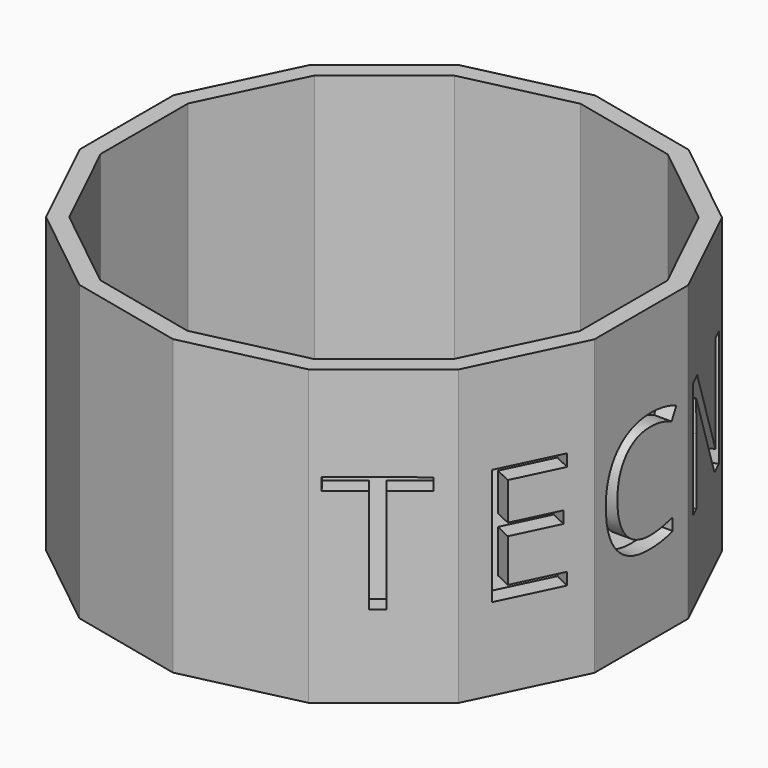
from build123d import *

# Parameters (mm, degrees)
F4_T          = -3
F5_TEXT_SIZE  = 27.7777777778
F6_DEPTH      = 25
F7_TEXT_SIZE  = 27.7777777778
F8_DEPTH      = 25
F9_TEXT_SIZE  = 27.7777777778
F10_DEPTH     = 25
F11_TEXT_SIZE = 27.7777777778
F12_DEPTH     = 25
F13_TEXT_SIZE = 27.7777777778
F14_DEPTH     = 25


# Not quite as in the source:
# - Text() gives the source's letters only with a copy of the font that has no kerning and outlines rounded to 1/6400 em; it was checked with that copy


with BuildPart() as f3:
    # F0 (on Top) → F3 section 0
    with BuildSketch(Plane.XY):
        Polygon((-19.4985582436, -40.4891733952), (0, -44.9395920743), (19.4985582436, -40.4891733952), (35.135187893, -28.019377358), (43.8128626753, -10), (43.8128626753, 10), (35.135187893, 28.019377358), (19.4985582436, 40.4891733952), (0, 44.9395920743), (-19.4985582436, 40.4891733952), (-35.135187893, 28.019377358), (-43.8128626753, 10), (-43.8128626753, -10), (-35.135187893, -28.019377358), align=None)
    # F2 (on offset) → F3 section 1
    with BuildSketch(Plane.XY.offset(50)):
        Polygon((19.4985582436, 40.4891733952), (0, 44.9395920743), (-19.4985582436, 40.4891733952), (-35.135187893, 28.019377358), (-43.8128626753, 10), (-43.8128626753, -10), (-35.135187893, -28.019377358), (-19.4985582436, -40.4891733952), (0, -44.9395920743), (19.4985582436, -40.4891733952), (35.135187893, -28.019377358), (43.8128626753, -10), (43.8128626753, 10), (35.135187893, 28.019377358), align=None)
    loft()

    # F4
    f4_openings = [f3.faces().sort_by_distance(p)[0] for p in [
        (0, 0, 50),
    ]]
    offset(amount=F4_T, openings=f4_openings)

    # F5 (on face) → F6 (cut)
    with BuildSketch(Plane(origin=(39.4740252842, -19.009688679, 0), x_dir=(0.4338837391, 0.9009688679, 0), z_dir=(0.9009688679, -0.4338837391, 0))):
        with Locations((-7.7907986111, 14)):
            Text('E', F5_TEXT_SIZE, font='Open Sans', text_align=(TextAlign.LEFT, TextAlign.BOTTOM))
    extrude(amount=-F6_DEPTH, mode=Mode.SUBTRACT)

    # F7 (on face) → F8 (cut)
    with BuildSketch(Plane.YZ.offset(43.8128626753)):
        with Locations((-9.2491319444, 14)):
            Text('C', F7_TEXT_SIZE, font='Open Sans', text_align=(TextAlign.LEFT, TextAlign.BOTTOM))
    extrude(amount=-F8_DEPTH, mode=Mode.SUBTRACT)

    # F9 (on face) → F10 (cut)
    with BuildSketch(Plane(origin=(39.4740252842, 19.009688679, 0), x_dir=(-0.4338837391, 0.9009688679, 0), z_dir=(0.9009688679, 0.4338837391, 0))):
        with Locations((-10.0086805556, 14)):
            Text('N', F9_TEXT_SIZE, font='Open Sans', text_align=(TextAlign.LEFT, TextAlign.BOTTOM))
    extrude(amount=-F10_DEPTH, mode=Mode.SUBTRACT)

    # F11 (on face) → F12 (cut)
    with BuildSketch(Plane(origin=(27.3168730683, 34.2542753766, 0), x_dir=(-0.7818314825, 0.6234898019, 0), z_dir=(0.6234898019, 0.7818314825, 0))):
        with Locations((-10.8702256944, 14)):
            Text('O', F11_TEXT_SIZE, font='Open Sans', text_align=(TextAlign.LEFT, TextAlign.BOTTOM))
    extrude(amount=-F12_DEPTH, mode=Mode.SUBTRACT)

    # F13 (on face) → F14 (cut)
    with BuildSketch(Plane(origin=(27.3168730683, -34.2542753766, 0), x_dir=(0.7818314825, 0.6234898019, 0), z_dir=(0.6234898019, -0.7818314825, 0))):
        with Locations((-8.4548611111, 14)):
            Text('T', F13_TEXT_SIZE, font='Open Sans', text_align=(TextAlign.LEFT, TextAlign.BOTTOM))
    extrude(amount=-F14_DEPTH, mode=Mode.SUBTRACT)


solid = f3.part
